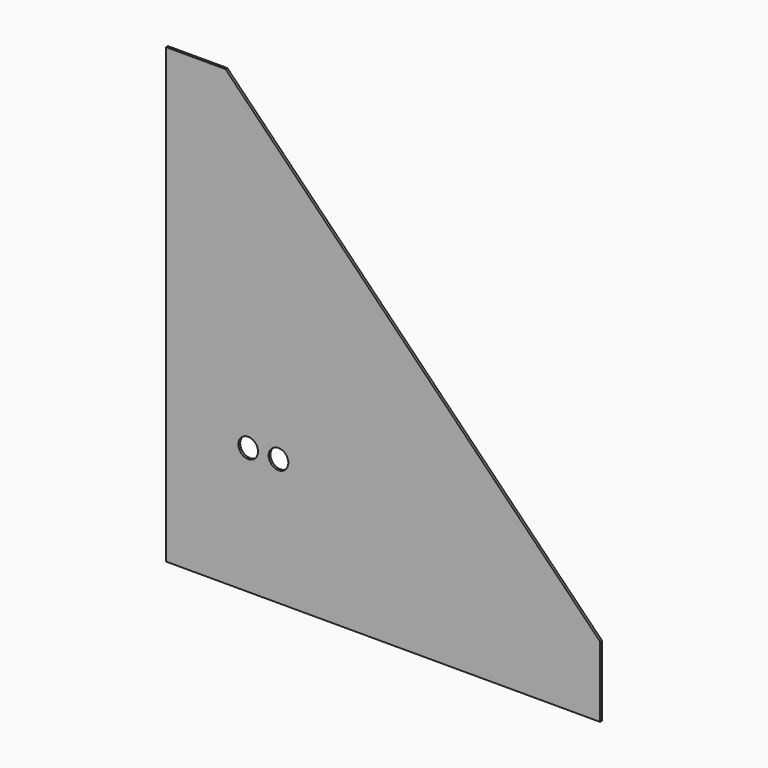
from build123d import *

# Parameters (mm, degrees)
F1_DEPTH = 6


with BuildPart() as f1:
    # F0 (on Front) → F1 (new body)
    with BuildSketch(Plane.XZ):
        with BuildLine():
            Line((-415, 600), (-572, 600))
            Line((-572, 600), (-572, -262))
            Line((-572, -262), (-381, -262))
            ThreePointArc((-381, -262), (-355, -236), (-329, -262))
            Line((-329, -262), (-301, -262))
            ThreePointArc((-301, -262), (-275, -236), (-249, -262))
            ThreePointArc((-249, -262), (-256.6152236891, -280.3847763109), (-275, -288))
            Line((-275, -288), (-275, -597))
            Line((-275, -597), (575, -597))
            Line((575, -597), (575, -410))
            Line((575, -410), (-415, 600))
        make_face()
        with BuildLine():
            Line((-381, -262), (-572, -262))
            Line((-572, -262), (-572, -597))
            Line((-572, -597), (-355, -597))
            Line((-355, -597), (-355, -288))
            ThreePointArc((-355, -288), (-373.3847763109, -280.3847763109), (-381, -262))
        make_face()
        with BuildLine():
            Line((-301, -262), (-329, -262))
            ThreePointArc((-329, -262), (-336.6152236891, -280.3847763109), (-355, -288))
            Line((-355, -288), (-355, -597))
            Line((-355, -597), (-275, -597))
            Line((-275, -597), (-275, -288))
            ThreePointArc((-275, -288), (-293.3847763109, -280.3847763109), (-301, -262))
        make_face()
    extrude(amount=F1_DEPTH)


solid = f1.part
